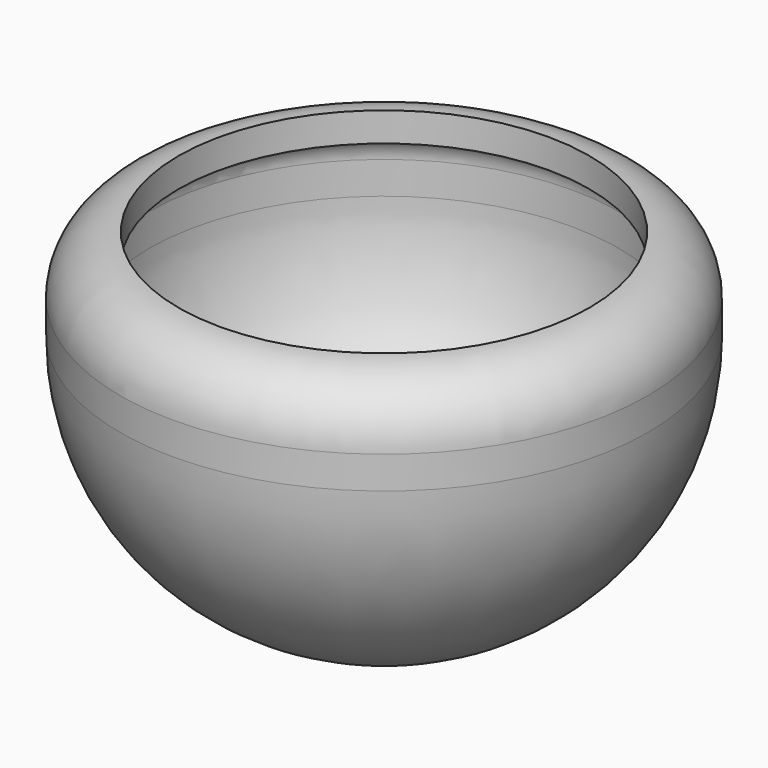
from build123d import *

# Parameters (mm, degrees)
F0_R     = 22.9481438371
F1_DEPTH = 29.972
F2_R     = 5.08
F3_R     = 22.0755688143
F4_T     = -2.54


# Not quite as in the source:
# - a shell that OpenCascade refuses in one call is made with other operations: the cavity is built on its own and cut out


with BuildPart() as f1:
    # F0 (on Top) → F1 (new body)
    with BuildSketch(Plane.XY):
        Circle(F0_R)
    extrude(amount=F1_DEPTH)

    # F2
    f2_edges = [f1.edges().sort_by_distance(p)[0] for p in [
        (-22.948144, 0, 29.972),
    ]]
    fillet(f2_edges, radius=F2_R)

    # F3
    f3_edges = [f1.edges().sort_by_distance(p)[0] for p in [
        (-22.948144, 0, 0),
    ]]
    fillet(f3_edges, radius=F3_R)

    # F4: a shell. OpenCascade refuses it in one call, so the cavity is built on its own and cut out:
    # the body offset inwards by the wall thickness, plus a prism from it out through each open face.
    f4_core = offset(f1.part, amount=F4_T, mode=Mode.PRIVATE)
    f4_exits = [f4_core.faces().sort_by_distance(p)[0] for p in [
        (0, 0, 27.432),
    ]]
    add(f4_core, mode=Mode.SUBTRACT)
    extrude(f4_exits, amount=-F4_T, mode=Mode.SUBTRACT)


solid = f1.part
